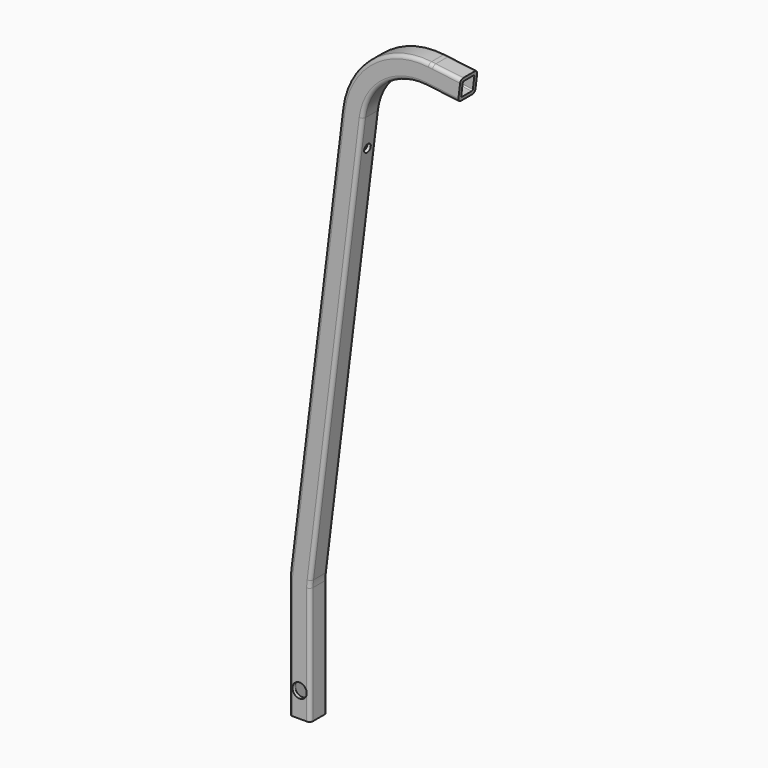
from build123d import *

# Parameters (mm, degrees)
F4_R      = 3.683
F5_DEPTH  = 334.01
F6_R      = 3.683
F7_DEPTH  = 25.4
F8_R      = 6.35
F9_DEPTH  = 9.4742
F11_DEPTH = 24.765
F12_R     = 6.35
F13_DEPTH = 12.446


# Not quite as in the source:
# - a feature names something its author has since deleted; it is built from what else it names


with BuildPart() as f2:
    # F2: sweep along a path in F0
    with BuildLine(Plane.XZ) as f2_path:
        Line((0, 0), (0, 104.902))
        ThreePointArc((0, 104.902), (0.1125182852, 108.5847531474), (0.4496534022, 112.2537681409))
        Line((0.4496534022, 112.2537681409), (46.8818732396, 490.4138519163))
        ThreePointArc((46.8818732396, 490.4138519163), (69.6174413383, 530.5988324867), (114.1089879783, 542.9374303731))
        Line((114.1089879783, 542.9374303731), (117.890588816, 542.4731081747))
    # F1 (on Top) → F2 (sweep)
    with BuildSketch(Plane.XY):
        with BuildLine():
            ThreePointArc((-9.525, -6.35), (-8.5950640303, -8.5950640303), (-6.35, -9.525))
            Line((-6.35, -9.525), (6.35, -9.525))
            ThreePointArc((6.35, -9.525), (8.5950640303, -8.5950640303), (9.525, -6.35))
            Line((9.525, -6.35), (9.525, 6.35))
            ThreePointArc((9.525, 6.35), (8.5950640303, 8.5950640303), (6.35, 9.525))
            Line((6.35, 9.525), (-6.35, 9.525))
            ThreePointArc((-6.35, 9.525), (-8.5950640303, 8.5950640303), (-9.525, 6.35))
            Line((-9.525, 6.35), (-9.525, -6.35))
        make_face()
        with BuildLine():
            Line((5.461, -6.477), (-5.461, -6.477))
            ThreePointArc((-5.461, -6.477), (-6.1794204897, -6.1794204897), (-6.477, -5.461))
            Line((-6.477, -5.461), (-6.477, 5.461))
            ThreePointArc((-6.477, 5.461), (-6.1794204897, 6.1794204897), (-5.461, 6.477))
            Line((-5.461, 6.477), (5.461, 6.477))
            ThreePointArc((5.461, 6.477), (6.1794204897, 6.1794204897), (6.477, 5.461))
            Line((6.477, 5.461), (6.477, -5.461))
            ThreePointArc((6.477, -5.461), (6.1794204897, -6.1794204897), (5.461, -6.477))
        make_face(mode=Mode.SUBTRACT)
    sweep(path=f2_path.line)

    # F4 (on Front) → F5 (cut, symmetric)
    with BuildSketch(Plane.XZ):
        with Locations((0, 22.225)):
            Circle(F4_R)
    extrude(amount=F5_DEPTH, both=True, mode=Mode.SUBTRACT)

    # F6 (on face) → F7 (cut)
    with BuildSketch(Plane(origin=(-22.5893491944, 0, 2.7736233219), x_dir=(0, -1, 0), z_dir=(-0.9925461516, 0, 0.1218693434))):
        with Locations((0, 464.5318445404)):
            Circle(F6_R)
    extrude(amount=-F7_DEPTH, mode=Mode.SUBTRACT)

    # F8 (on face) → F9 (cut)
    with BuildSketch(Plane(origin=(-22.5893491944, 0, 2.7736233219), x_dir=(0, -1, 0), z_dir=(-0.9925461516, 0, 0.1218693434))):
        with Locations((0, 464.5318445404)):
            Circle(F8_R)
    extrude(amount=-F9_DEPTH, mode=Mode.SUBTRACT)

    # F10 (on face) → F11 (join)
    with BuildSketch(Plane(origin=(50.5216003355, 0, -6.2032725133), x_dir=(0, 1, 0), z_dir=(0.9925461516, 0, -0.1218693434))):
        with BuildLine():
            ThreePointArc((9.525, 559.1468445404), (8.5950640303, 561.3919085707), (6.35, 562.3218445404))
            Line((6.35, 562.3218445404), (-6.35, 562.3218445404))
            ThreePointArc((-6.35, 562.3218445404), (-8.5950640303, 561.3919085707), (-9.525, 559.1468445404))
            Line((-9.525, 559.1468445404), (-9.525, 546.4468445404))
            ThreePointArc((-9.525, 546.4468445404), (-8.5950640303, 544.2017805101), (-6.35, 543.2718445404))
            Line((-6.35, 543.2718445404), (6.35, 543.2718445404))
            ThreePointArc((6.35, 543.2718445404), (8.5950640303, 544.2017805101), (9.525, 546.4468445404))
            Line((9.525, 546.4468445404), (9.525, 559.1468445404))
        make_face()
        with BuildLine():
            ThreePointArc((-6.477, 558.2578445404), (-6.1794204897, 558.9762650301), (-5.461, 559.2738445404))
            Line((-5.461, 559.2738445404), (5.461, 559.2738445404))
            ThreePointArc((5.461, 559.2738445404), (6.1794204897, 558.9762650301), (6.477, 558.2578445404))
            Line((6.477, 558.2578445404), (6.477, 547.3358445404))
            ThreePointArc((6.477, 547.3358445404), (6.1794204897, 546.6174240507), (5.461, 546.3198445404))
            Line((5.461, 546.3198445404), (-5.461, 546.3198445404))
            ThreePointArc((-5.461, 546.3198445404), (-6.1794204897, 546.6174240507), (-6.477, 547.3358445404))
            Line((-6.477, 547.3358445404), (-6.477, 558.2578445404))
        make_face(mode=Mode.SUBTRACT)
    extrude(amount=F11_DEPTH)

    # F12 (on face) → F13 (cut)
    with BuildSketch(Plane.XZ.offset(9.525)):
        with Locations((0, 22.225)):
            Circle(F12_R)
    extrude(amount=-F13_DEPTH, mode=Mode.SUBTRACT)


solid = f2.part
